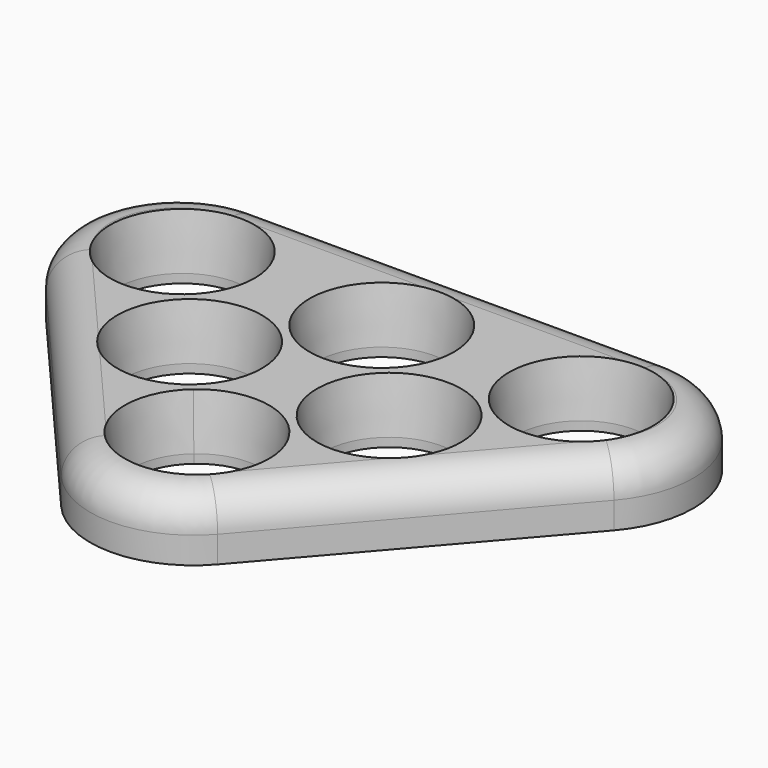
from build123d import *

# Parameters (mm, degrees)
F0_R         = 9.3483634699
F1_DEPTH     = 8.89
F2_R         = 14.8297125388
F3_SIZE2     = 1.016
F3_SIZE      = 7.62
F3_2_SIZE2   = 1.016
F3_2_SIZE    = 7.62
F3_3_SIZE2   = 1.016
F3_3_SIZE    = 7.62
F3_4_SIZE2   = 1.016
F3_4_SIZE    = 7.62
F3_5_SIZE2   = 1.016
F3_5_SIZE    = 7.62
F3_6_SIZE2   = 1.016
F3_6_SIZE    = 7.62
F4_T1_DEPTH  = 45.1686724369
F4_T3_DEPTH  = 45.1686724369
F4_T5_DEPTH  = 59.0377910967
F4_T8_ANGLE  = 130.8079672241
F4_T10_ANGLE = 98.3840655518
F4_T12_ANGLE = 130.8079672241


# Not quite as in the source:
# - a fillet or chamfer that OpenCascade refuses, or shapes differently, is made with other operations: its cross-section is extruded or revolved along the edge and cut away or added
# - a feature names something its author has since deleted; it is built from what else it names


with BuildPart() as f1:
    # F0 (on Top) → F1 (new body)
    with BuildSketch(Plane.XY):
        Polygon((-61.9157478895, 31.8151319193), (-35.3605267654, 1.0592594085), (0, -39.8947905701), (61.9157478895, 31.8151319193), (0, 31.8151319193), align=None)
        with BuildLine():
            ThreePointArc((-6.1093972864, -9.4993164637), (3.8909531705, -8.0749917446), (9.3483634699, -16.5751319193))
            ThreePointArc((9.3483634699, -16.5751319193), (-3.8909531705, -25.075272094), (-6.1093972864, -9.4993164637))
        make_face(mode=Mode.SUBTRACT)
        with Locations((-14.3112926848, 0)):
            Circle(F0_R, mode=Mode.SUBTRACT)
        with Locations((-28.6225853696, 16.5751319193)):
            Circle(F0_R, mode=Mode.SUBTRACT)
        with Locations((14.3112926848, 0)):
            Circle(F0_R, mode=Mode.SUBTRACT)
        with Locations((0, 16.5751319193)):
            Circle(F0_R, mode=Mode.SUBTRACT)
        with Locations((28.6225853696, 16.5751319193)):
            Circle(F0_R, mode=Mode.SUBTRACT)
    extrude(amount=F1_DEPTH)

    # F2
    f2_edges = [f1.edges().sort_by_distance(p)[0] for p in [
        (0, -39.894791, 4.445),
        (-61.915748, 31.815132, 4.445),
        (61.915748, 31.815132, 4.445),
    ]]
    fillet(f2_edges, radius=F2_R)

    # F3
    f3_edges = [f1.edges().sort_by_distance(p)[0] for p in [
        (-37.970949, 16.575132, 8.89),
    ]]
    f3_side = f1.faces().sort_by_distance((-37.970949, 16.575132, 4.445))[0]
    chamfer(f3_edges, length=F3_SIZE, length2=F3_SIZE2, reference=f3_side)

    # F3#2
    f3_2_edges = [f1.edges().sort_by_distance(p)[0] for p in [
        (-23.659656, 0, 8.89),
    ]]
    f3_2_side = f1.faces().sort_by_distance((-23.659656, 0, 4.445))[0]
    chamfer(f3_2_edges, length=F3_2_SIZE, length2=F3_2_SIZE2, reference=f3_2_side)

    # F3#3
    f3_3_edges = [f1.edges().sort_by_distance(p)[0] for p in [
        (-9.348363, 16.575132, 8.89),
    ]]
    f3_3_side = f1.faces().sort_by_distance((-9.348363, 16.575132, 4.445))[0]
    chamfer(f3_3_edges, length=F3_3_SIZE, length2=F3_3_SIZE2, reference=f3_3_side)

    # F3#4
    f3_4_edges = [f1.edges().sort_by_distance(p)[0] for p in [
        (4.962929, 0, 8.89),
    ]]
    f3_4_side = f1.faces().sort_by_distance((4.962929, 0, 4.445))[0]
    chamfer(f3_4_edges, length=F3_4_SIZE, length2=F3_4_SIZE2, reference=f3_4_side)

    # F3#5
    f3_5_edges = [f1.edges().sort_by_distance(p)[0] for p in [
        (19.274222, 16.575132, 8.89),
    ]]
    f3_5_side = f1.faces().sort_by_distance((19.274222, 16.575132, 4.445))[0]
    chamfer(f3_5_edges, length=F3_5_SIZE, length2=F3_5_SIZE2, reference=f3_5_side)

    # F3#6
    f3_6_edges = [f1.edges().sort_by_distance(p)[0] for p in [
        (6.109397, -23.650947, 8.89),
    ]]
    f3_6_side = f1.faces().sort_by_distance((6.109397, -23.650947, 4.445))[0]
    chamfer(f3_6_edges, length=F3_6_SIZE, length2=F3_6_SIZE2, reference=f3_6_side)

    # F4: fillet of radius 5.08 on 6 edges, made by hand

    # F4_s2 → F4_t1 (cut)
    with BuildSketch(Plane(origin=(8.5095443903, -9.8556310704, 0), x_dir=(0, 0, 1), z_dir=(-0.6535258611, 0.7569041874, 0))):
        with BuildLine():
            ThreePointArc((8.89, -20.9922773601), (7.4021024484, -24.5843798086), (3.81, -26.0722773601))
            Line((3.81, -26.0722773601), (8.89, -26.0722773601))
            Line((8.89, -26.0722773601), (8.89, -20.9922773601))
        make_face()
    extrude(amount=F4_T1_DEPTH, mode=Mode.SUBTRACT)

    # F4_s4 → F4_t3 (cut)
    with BuildSketch(Plane(origin=(-8.5095443903, -9.8556310704, 0), x_dir=(0, 0, 1), z_dir=(0.6535258611, 0.7569041874, 0))):
        with BuildLine():
            ThreePointArc((8.89, 20.9922773601), (7.4021024484, 24.5843798086), (3.81, 26.0722773601))
            Line((3.81, 26.0722773601), (8.89, 26.0722773601))
            Line((8.89, 26.0722773601), (8.89, 20.9922773601))
        make_face()
    extrude(amount=F4_T3_DEPTH, mode=Mode.SUBTRACT)

    # F4_s6 → F4_t5 (cut)
    with BuildSketch(Plane.YZ.offset(-29.5188955483)):
        with BuildLine():
            ThreePointArc((26.7351319193, 8.89), (30.3272343677, 7.4021024484), (31.8151319193, 3.81))
            Line((31.8151319193, 3.81), (31.8151319193, 8.89))
            Line((31.8151319193, 8.89), (26.7351319193, 8.89))
        make_face()
    extrude(amount=F4_T5_DEPTH, mode=Mode.SUBTRACT)

    # F4_s7 → F4_t8 (revolve, cut)
    with BuildSketch(Plane.YZ.offset(-29.5188955483)):
        with BuildLine():
            ThreePointArc((26.7351319193, 8.89), (30.3272343677, 7.4021024484), (31.8151319193, 3.81))
            Line((31.8151319193, 3.81), (31.8151319193, 8.89))
            Line((31.8151319193, 8.89), (26.7351319193, 8.89))
        make_face()
    revolve(axis=Axis((-29.5188955483, 16.9854193804, 8.89), (0, 0, 1)), revolution_arc=F4_T8_ANGLE, mode=Mode.SUBTRACT)

    # F4_s9 → F4_t10 (revolve, cut)
    with BuildSketch(Plane(origin=(8.5095443903, -9.8556310704, 0), x_dir=(0, 0, 1), z_dir=(-0.6535258611, 0.7569041874, 0))):
        with BuildLine():
            ThreePointArc((8.89, -20.9922773601), (7.4021024484, -24.5843798086), (3.81, -26.0722773601))
            Line((3.81, -26.0722773601), (8.89, -26.0722773601))
            Line((8.89, -26.0722773601), (8.89, -20.9922773601))
        make_face()
    revolve(axis=Axis((0, -17.202937926, 8.89), (0, 0, 1)), revolution_arc=F4_T10_ANGLE, mode=Mode.SUBTRACT)

    # F4_s11 → F4_t12 (revolve, cut)
    with BuildSketch(Plane.YZ.offset(29.5188955483)):
        with BuildLine():
            ThreePointArc((26.7351319193, 8.89), (30.3272343677, 7.4021024484), (31.8151319193, 3.81))
            Line((31.8151319193, 3.81), (31.8151319193, 8.89))
            Line((31.8151319193, 8.89), (26.7351319193, 8.89))
        make_face()
    revolve(axis=Axis((29.5188955483, 16.9854193804, 8.89), (0, 0, -1)), revolution_arc=F4_T12_ANGLE, mode=Mode.SUBTRACT)


solid = f1.part
